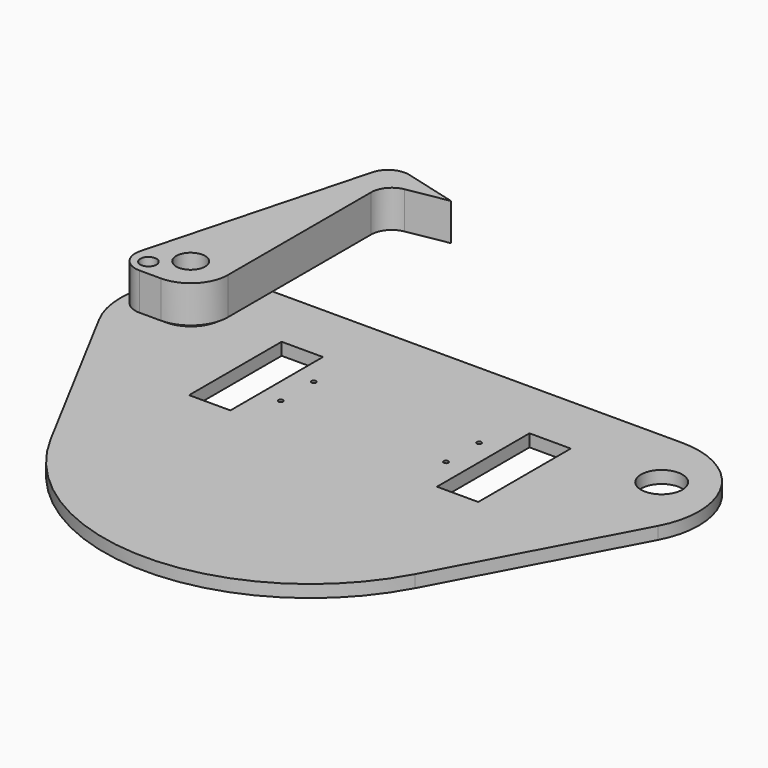
from build123d import *

# Parameters (mm, degrees)
F0_W           = 50
F0_H           = 140
F1_DEPTH       = 15
F2_R           = 25
F3_DEPTH       = 15.001
F4_R           = 25
F4_R_2         = 17.5
F5_DEPTH       = 15
F6_R           = 37.5
F6_R_2         = 17.5
F7_DEPTH       = 5
F9_D           = 5.5
F9_CBORE_D     = 9.75
F9_CBORE_DEPTH = 5
F10_R          = 45
F10_R_2        = 17.5
F11_DEPTH      = 45
F12_R          = 17.5
F13_DEPTH      = 45
F14_R          = 9.7715412821
F15_DEPTH      = 65.001
F16_R          = 25


with BuildPart() as f1:
    # F0 (on Top) → F1 (new body)
    with BuildSketch(Plane.XY):
        with BuildLine():
            Line((250, 0), (-250, 0))
            ThreePointArc((-250, 0), (-335.7492925713, -48.5504244572), (-338.2352941176, -147.0588235294))
            Line((-338.2352941176, -147.0588235294), (-220.5882352941, -367.6470588235))
            ThreePointArc((-220.5882352941, -367.6470588235), (0, -500), (220.5882352941, -367.6470588235))
            Line((220.5882352941, -367.6470588235), (338.2352941176, -147.0588235294))
            ThreePointArc((338.2352941176, -147.0588235294), (335.7492925713, -48.5504244572), (250, 0))
        make_face()
        with Locations((-150, -145)):
            Rectangle(F0_W, F0_H, mode=Mode.SUBTRACT)
        with Locations((150, -145)):
            Rectangle(F0_W, F0_H, mode=Mode.SUBTRACT)
    extrude(amount=F1_DEPTH)

    # F2 (on face) → F3 (cut, through all)
    with BuildSketch(Plane.XY.offset(15)):
        with Locations((-285, -75)):
            Circle(F2_R)
        with Locations((285, -75)):
            Circle(F2_R)
    extrude(amount=-F3_DEPTH, mode=Mode.SUBTRACT)

    # F9 (through all)
    with Locations(Plane(origin=(0, 0, 0), x_dir=(1, 0, 0), z_dir=(0, 0, -1))):
        with Locations((-100, 120), (-100, 170), (100, 120), (100, 170)):
            CounterBoreHole(F9_D / 2, F9_CBORE_D / 2, F9_CBORE_DEPTH)


with BuildPart() as f5:
    # F4 (on face) → F5 (new body)
    with BuildSketch(Plane.XY.offset(15)):
        with Locations((-285, -75)):
            Circle(F4_R)
        with Locations((-285, -75)):
            Circle(F4_R_2, mode=Mode.SUBTRACT)
    extrude(amount=-F5_DEPTH)

    # F6 (on face) → F7 (join)
    with BuildSketch(Plane.XY.offset(15)):
        with Locations((-285, -75)):
            Circle(F6_R)
        with Locations((-285, -75)):
            Circle(F6_R_2, mode=Mode.SUBTRACT)
    extrude(amount=F7_DEPTH)


with BuildPart() as f11:
    # F10 (on face) → F11 (new body)
    with BuildSketch(Plane.XY.offset(20)):
        with Locations((-285, -75)):
            Circle(F10_R)
        with Locations((-285, -75)):
            Circle(F10_R_2, mode=Mode.SUBTRACT)
    extrude(amount=F11_DEPTH)

    # F12 (on face) → F13 (join, through all)
    with BuildSketch(Plane(origin=(0, 0, 20), x_dir=(1, 0, 0), z_dir=(0, 0, -1))):
        with BuildLine():
            Line((-240, -162.6571113504), (-240, 75))
            ThreePointArc((-240, 75), (-253.1801948466, 106.8198051534), (-285, 120))
            Line((-285, 120), (-343.6451417779, 120))
            Line((-343.6451417779, 120), (-258.2631229006, -198.6500325027))
            Line((-258.2631229006, -198.6500325027), (-170, -175))
            Line((-170, -175), (-240, -162.6571113504))
        make_face()
        with Locations((-285, 75)):
            Circle(F12_R, mode=Mode.SUBTRACT)
    extrude(amount=-F13_DEPTH)

    # F14 (on face) → F15 (cut, through all)
    with BuildSketch(Plane.XY.offset(65)):
        with Locations((-315.6417777248, -100.7115043875)):
            Circle(F14_R)
    extrude(amount=-F15_DEPTH, mode=Mode.SUBTRACT)

    # F16
    f16_edges = [f11.edges().sort_by_distance(p)[0] for p in [
        (-240, 162.657111, 42.5),
        (-258.263123, 198.650033, 42.5),
        (-343.645142, -120, 42.5),
    ]]
    fillet(f16_edges, radius=F16_R)


solid = Compound([f1.part, f5.part, f11.part])
